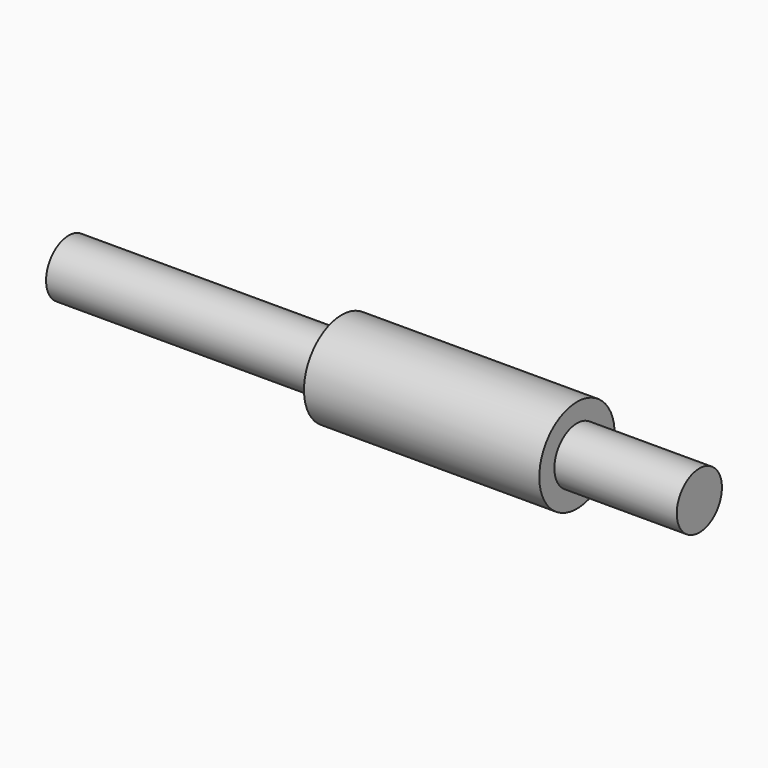
from build123d import *

# Parameters (mm, degrees)
F0_W   = 23
F0_H   = 3
F0_W_2 = 6
F0_W_3 = 13


# Not quite as in the source:
# - a feature names something its author has since deleted; it is built from what else it names


with BuildPart() as f1:
    # F0 (on Front) → F1 (revolve)
    with BuildSketch(Plane.XZ):
        Polygon((25, 5), (0, 5), (0, 3), (0, 0), (25, 0), (25, 3), align=None)
        with Locations((-11.5, 1.5)):
            Rectangle(F0_W, F0_H)
        with Locations((-26, 1.5)):
            Rectangle(F0_W_2, F0_H)
        with Locations((31.5, 1.5)):
            Rectangle(F0_W_3, F0_H)
    revolve(axis=Axis((1, 0, 0), (1, 0, 0)))


solid = f1.part
